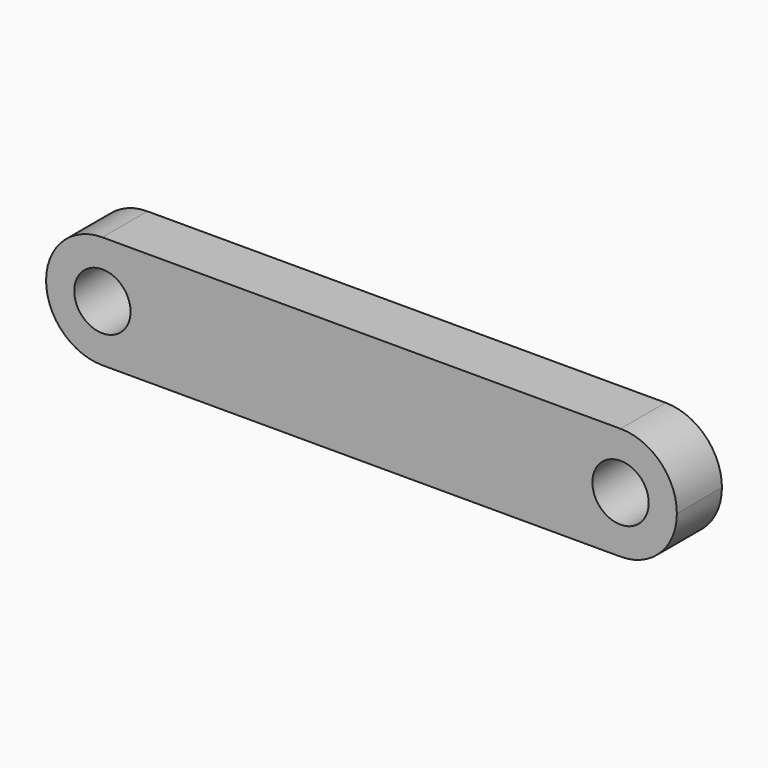
from build123d import *

# Parameters (mm, degrees)
F0_W     = 71.12
F0_H     = 12.7
F1_DEPTH = 6.35
F2_R     = 6.34999
F3_R     = 3.175
F4_DEPTH = 6.351


# Not quite as in the source:
# - a fillet or chamfer is up to 0.001 mm smaller than in the source, because OpenCascade refuses the exact size


with BuildPart() as f1:
    # F0 (on Front) → F1 (new body)
    with BuildSketch(Plane.XZ):
        with Locations((35.56, 6.35)):
            Rectangle(F0_W, F0_H)
    extrude(amount=F1_DEPTH)

    # F2 (radius 6.35 in the source; OpenCascade refuses exactly that, so slightly less here)
    f2_edges = [f1.edges().sort_by_distance(p)[0] for p in [
        (71.12, -3.175, 12.7),
        (71.12, -3.175, 0),
        (0, -3.175, 12.7),
        (0, -3.175, 0),
    ]]
    fillet(f2_edges, radius=F2_R)

    # F3 (on face) → F4 (cut, through all)
    with BuildSketch(Plane.XZ.offset(6.35)):
        with Locations((6.35, 6.35)):
            Circle(F3_R)
        with Locations((64.77, 6.35)):
            Circle(F3_R)
    extrude(amount=-F4_DEPTH, mode=Mode.SUBTRACT)


solid = f1.part
